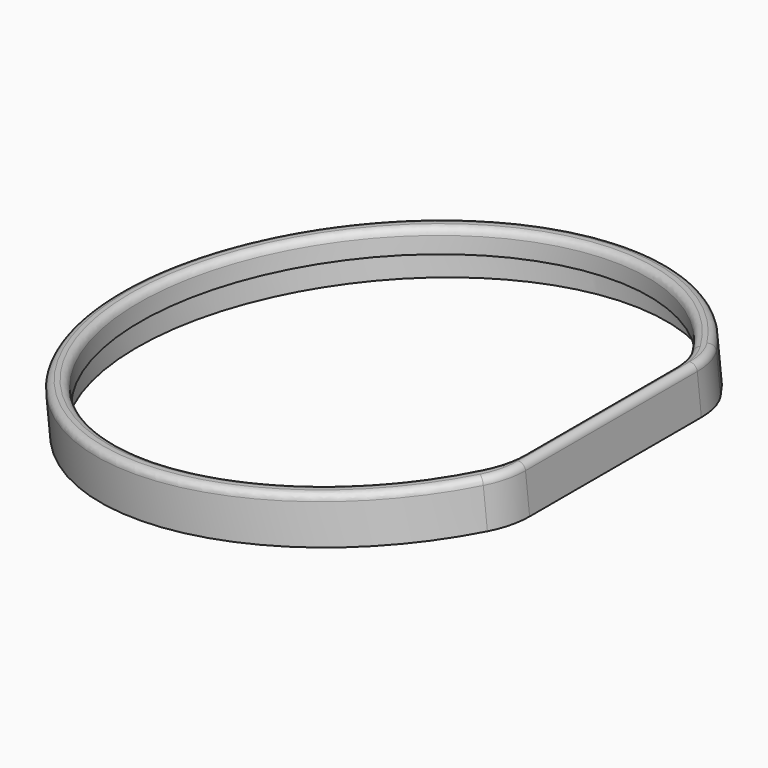
from build123d import *

# Parameters (mm, degrees)
F3_DEPTH     = 5
F4_DEPTH     = 5
F5_R         = 15
F6_T1_DEPTH  = 46.5006688801
F6_T3_DEPTH  = 40.6046915678
F6_T6_ANGLE  = 292.774155129
F6_T8_ANGLE  = 295.4108576805
F6_T10_ANGLE = 33.6129224355
F6_T12_ANGLE = 33.6129224355
F6_T14_ANGLE = 32.2945711597
F6_T16_ANGLE = 32.2945711597


# Not quite as in the source:
# - a fillet or chamfer that OpenCascade refuses, or shapes differently, is made with other operations: its cross-section is extruded or revolved along the edge and cut away or added


with BuildPart() as f3:
    # F2 (on line) → F3 (new body)
    with BuildSketch(Plane(origin=(-1.0990247565, 0, 10.4565220775), x_dir=(0.9945218954, 0, 0.1045284633), z_dir=(-0.1045284633, 0, 0.9945218954))):
        with BuildLine():
            add(Edge.make_bspline(
                [(48.8576467338, 27.4245012731), (32.937142649, 55.0146028399), (1, 55.0146028399)],
                knots=[3.6634544085, 3.6634544085, 3.6634544085, 4.7123889804, 4.7123889804, 4.7123889804], degree=2, weights=[1, 0.865590822, 1]))
            add(Edge.make_bspline(
                [(49.9774491412, 25.3853808752), (49.4391671103, 26.4167312826), (48.8576467338, 27.4245012731)],
                knots=[3.6211988828, 3.6211988828, 3.6211988828, 3.6634544085, 3.6634544085, 3.6634544085], degree=2, weights=[1, 0.9997768171, 1]))
            Line((49.9774491412, 25.3853808752), (49.9774491412, 27.409023648))
            ThreePointArc((49.9774491412, 27.409023648), (-57, 0), (49.9774491412, -27.409023648))
            Line((49.9774491412, -27.409023648), (49.9774491412, -25.3853808752))
            add(Edge.make_bspline(
                [(48.8576467338, -27.4245012731), (49.4391671103, -26.4167312826), (49.9774491412, -25.3853808752)],
                knots=[2.6197308987, 2.6197308987, 2.6197308987, 2.6619864244, 2.6619864244, 2.6619864244], degree=2, weights=[1, 0.9997768171, 1]))
            add(Edge.make_bspline(
                [(1, 55.0146028399), (-94.7155099565, 55.0146028399), (-46.785780422, -27.5486703855), (1.1439491125, -110.1119436109), (48.8576467338, -27.4245012731)],
                knots=[4.7123889804, 4.7123889804, 4.7123889804, 6.8076525931, 6.8076525931, 8.9029162059, 8.9029162059, 8.9029162059], degree=2, weights=[1, 0.4996238769, 1, 0.4996238769, 1]))
        make_face()
        with BuildLine():
            ThreePointArc((47.121873477, -24.2596174747), (-53, 0), (47.121873477, 24.2596174747))
            ThreePointArc((47.121873477, 24.2596174747), (48.0257660969, 22.4170870276), (48.8576467338, 20.540943397))
            Line((48.8576467338, 20.540943397), (48.8576467338, 27.4245012731))
            add(Edge.make_bspline(
                [(48.8576467338, 27.4245012731), (32.937142649, 55.0146028399), (1, 55.0146028399)],
                knots=[3.6634544085, 3.6634544085, 3.6634544085, 4.7123889804, 4.7123889804, 4.7123889804], degree=2, weights=[1, 0.865590822, 1]))
            add(Edge.make_bspline(
                [(1, 55.0146028399), (-94.7155099565, 55.0146028399), (-46.785780422, -27.5486703855), (1.1439491125, -110.1119436109), (48.8576467338, -27.4245012731)],
                knots=[4.7123889804, 4.7123889804, 4.7123889804, 6.8076525931, 6.8076525931, 8.9029162059, 8.9029162059, 8.9029162059], degree=2, weights=[1, 0.4996238769, 1, 0.4996238769, 1]))
            Line((48.8576467338, -27.4245012731), (48.8576467338, -20.540943397))
            ThreePointArc((48.8576467338, -20.540943397), (48.0257660969, -22.4170870276), (47.121873477, -24.2596174747))
        make_face()
        with BuildLine():
            ThreePointArc((48.8576467338, 20.540943397), (48.0257660969, 22.4170870276), (47.121873477, 24.2596174747))
            Line((47.121873477, 24.2596174747), (47.121873477, -24.2596174747))
            ThreePointArc((47.121873477, -24.2596174747), (48.0257660969, -22.4170870276), (48.8576467338, -20.540943397))
            Line((48.8576467338, -20.540943397), (48.8576467338, 20.540943397))
        make_face()
        with BuildLine():
            ThreePointArc((49.9774491412, 17.6424084902), (49.4387946891, 19.0998842848), (48.8576467338, 20.540943397))
            Line((48.8576467338, 20.540943397), (48.8576467338, -20.540943397))
            ThreePointArc((48.8576467338, -20.540943397), (49.4387946891, -19.0998842848), (49.9774491412, -17.6424084902))
            Line((49.9774491412, -17.6424084902), (49.9774491412, 17.6424084902))
        make_face()
        with BuildLine():
            Line((48.8576467338, 27.4245012731), (48.8576467338, 20.540943397))
            ThreePointArc((48.8576467338, 20.540943397), (49.4387946891, 19.0998842848), (49.9774491412, 17.6424084902))
            Line((49.9774491412, 17.6424084902), (49.9774491412, 25.3853808752))
            add(Edge.make_bspline(
                [(49.9774491412, 25.3853808752), (49.4391671103, 26.4167312826), (48.8576467338, 27.4245012731)],
                knots=[3.6211988828, 3.6211988828, 3.6211988828, 3.6634544085, 3.6634544085, 3.6634544085], degree=2, weights=[1, 0.9997768171, 1]))
        make_face()
        with BuildLine():
            ThreePointArc((49.9774491412, -17.6424084902), (49.4387946891, -19.0998842848), (48.8576467338, -20.540943397))
            Line((48.8576467338, -20.540943397), (48.8576467338, -27.4245012731))
            add(Edge.make_bspline(
                [(48.8576467338, -27.4245012731), (49.4391671103, -26.4167312826), (49.9774491412, -25.3853808752)],
                knots=[2.6197308987, 2.6197308987, 2.6197308987, 2.6619864244, 2.6619864244, 2.6619864244], degree=2, weights=[1, 0.9997768171, 1]))
            Line((49.9774491412, -25.3853808752), (49.9774491412, -17.6424084902))
        make_face()
    extrude(amount=F3_DEPTH)

    # F2 (on line) → F4 (join)
    with BuildSketch(Plane(origin=(-1.0990247565, 0, 10.4565220775), x_dir=(0.9945218954, 0, 0.1045284633), z_dir=(-0.1045284633, 0, 0.9945218954))):
        with BuildLine():
            add(Edge.make_bspline(
                [(48.8576467338, 27.4245012731), (32.937142649, 55.0146028399), (1, 55.0146028399)],
                knots=[3.6634544085, 3.6634544085, 3.6634544085, 4.7123889804, 4.7123889804, 4.7123889804], degree=2, weights=[1, 0.865590822, 1]))
            add(Edge.make_bspline(
                [(49.9774491412, 25.3853808752), (49.4391671103, 26.4167312826), (48.8576467338, 27.4245012731)],
                knots=[3.6211988828, 3.6211988828, 3.6211988828, 3.6634544085, 3.6634544085, 3.6634544085], degree=2, weights=[1, 0.9997768171, 1]))
            Line((49.9774491412, 25.3853808752), (49.9774491412, 27.409023648))
            ThreePointArc((49.9774491412, 27.409023648), (-57, 0), (49.9774491412, -27.409023648))
            Line((49.9774491412, -27.409023648), (49.9774491412, -25.3853808752))
            add(Edge.make_bspline(
                [(48.8576467338, -27.4245012731), (49.4391671103, -26.4167312826), (49.9774491412, -25.3853808752)],
                knots=[2.6197308987, 2.6197308987, 2.6197308987, 2.6619864244, 2.6619864244, 2.6619864244], degree=2, weights=[1, 0.9997768171, 1]))
            add(Edge.make_bspline(
                [(1, 55.0146028399), (-94.7155099565, 55.0146028399), (-46.785780422, -27.5486703855), (1.1439491125, -110.1119436109), (48.8576467338, -27.4245012731)],
                knots=[4.7123889804, 4.7123889804, 4.7123889804, 6.8076525931, 6.8076525931, 8.9029162059, 8.9029162059, 8.9029162059], degree=2, weights=[1, 0.4996238769, 1, 0.4996238769, 1]))
        make_face()
        with BuildLine():
            ThreePointArc((49.9774491412, -17.6424084902), (49.4387946891, -19.0998842848), (48.8576467338, -20.540943397))
            Line((48.8576467338, -20.540943397), (48.8576467338, -27.4245012731))
            add(Edge.make_bspline(
                [(48.8576467338, -27.4245012731), (49.4391671103, -26.4167312826), (49.9774491412, -25.3853808752)],
                knots=[2.6197308987, 2.6197308987, 2.6197308987, 2.6619864244, 2.6619864244, 2.6619864244], degree=2, weights=[1, 0.9997768171, 1]))
            Line((49.9774491412, -25.3853808752), (49.9774491412, -17.6424084902))
        make_face()
        with BuildLine():
            Line((48.8576467338, 27.4245012731), (48.8576467338, 20.540943397))
            ThreePointArc((48.8576467338, 20.540943397), (49.4387946891, 19.0998842848), (49.9774491412, 17.6424084902))
            Line((49.9774491412, 17.6424084902), (49.9774491412, 25.3853808752))
            add(Edge.make_bspline(
                [(49.9774491412, 25.3853808752), (49.4391671103, 26.4167312826), (48.8576467338, 27.4245012731)],
                knots=[3.6211988828, 3.6211988828, 3.6211988828, 3.6634544085, 3.6634544085, 3.6634544085], degree=2, weights=[1, 0.9997768171, 1]))
        make_face()
        with BuildLine():
            ThreePointArc((49.9774491412, 17.6424084902), (49.4387946891, 19.0998842848), (48.8576467338, 20.540943397))
            Line((48.8576467338, 20.540943397), (48.8576467338, -20.540943397))
            ThreePointArc((48.8576467338, -20.540943397), (49.4387946891, -19.0998842848), (49.9774491412, -17.6424084902))
            Line((49.9774491412, -17.6424084902), (49.9774491412, 17.6424084902))
        make_face()
    extrude(amount=-F4_DEPTH)

    # F5
    f5_edges = [f3.edges().sort_by_distance(p)[0] for p in [
        (45.503389, 24.259617, 17.868404),
        (47.752296, 27.424501, 13.077232),
        (48.604643, -27.409024, 15.680588),
        (48.604643, 27.409024, 15.680588),
        (47.752296, -27.424501, 13.077232),
        (45.503389, -24.259617, 17.868404),
    ]]
    fillet(f5_edges, radius=F5_R)

    # F6: fillet of radius 1.5 on 8 edges, made by hand

    # F6_s2 → F6_t1 (cut)
    with BuildSketch(Plane.XZ.offset(-23.25033444)):
        with BuildLine():
            ThreePointArc((48.2387930677, 19.161414668), (47.6909908112, 20.1703409153), (46.5902175297, 20.4964048162))
            Line((46.5902175297, 20.4964048162), (48.0820003728, 20.6531975111))
            Line((48.0820003728, 20.6531975111), (48.2387930677, 19.161414668))
        make_face()
    extrude(amount=F6_T1_DEPTH, mode=Mode.SUBTRACT)

    # F6_s4 → F6_t3 (cut)
    with BuildSketch(Plane.XZ.offset(-20.3023457839)):
        with BuildLine():
            ThreePointArc((46.7338506938, 20.5115012701), (45.7249244466, 19.9636990136), (45.3988605457, 18.8629257321))
            Line((45.3988605457, 18.8629257321), (45.2420678508, 20.3547085752))
            Line((45.2420678508, 20.3547085752), (46.7338506938, 20.5115012701))
        make_face()
    extrude(amount=F6_T3_DEPTH, mode=Mode.SUBTRACT)

    # F6_s5 → F6_t6 (revolve, cut)
    with BuildSketch(Plane(origin=(0, 0, 0), x_dir=(0.8341941601, 0.5514708544, 0), z_dir=(0.5505468256, -0.8327964081, 0.0578648031))):
        with BuildLine():
            ThreePointArc((53.9358200017, 20.2944629237), (55.0307493385, 19.9492829243), (55.5609021792, 18.930971847))
            Line((55.5609021792, 18.930971847), (55.4301066288, 20.4252584742))
            Line((55.4301066288, 20.4252584742), (53.9358200017, 20.2944629237))
        make_face()
    revolve(axis=Axis((-1.6216670728, 0, 15.4291315543), (-0.1045284633, 0, 0.9945218954)), revolution_arc=F6_T6_ANGLE, mode=Mode.SUBTRACT)

    # F6_s7 → F6_t8 (revolve, cut)
    with BuildSketch(Plane(origin=(0, 0, 0), x_dir=(-0.8466337525, 0.5321759946, 0), z_dir=(0.5313454581, 0.8453124599, 0.055846658))):
        with BuildLine():
            ThreePointArc((-52.9132065092, 20.2763527671), (-51.8955883279, 19.7448711382), (-51.5518378751, 18.6494921577))
            Line((-51.5518378751, 18.6494921577), (-51.4190918875, 20.1436067794))
            Line((-51.4190918875, 20.1436067794), (-52.9132065092, 20.2763527671))
        make_face()
    revolve(axis=Axis((-1.6216670728, 0, 15.4291315543), (0.1045284633, 0, -0.9945218954)), revolution_arc=F6_T8_ANGLE, mode=Mode.SUBTRACT)

    # F6_s9 → F6_t10 (revolve, cut)
    with BuildSketch(Plane.XZ.offset(23.25033444)):
        with BuildLine():
            ThreePointArc((46.5902175297, 20.4964048162), (47.6909908112, 20.1703409153), (48.2387930677, 19.161414668))
            Line((48.2387930677, 19.161414668), (48.0820003728, 20.6531975111))
            Line((48.0820003728, 20.6531975111), (46.5902175297, 20.4964048162))
        make_face()
    revolve(axis=Axis((33.1641719422, -23.25033444, 19.0852705621), (0.1045284633, 0, -0.9945218954)), revolution_arc=F6_T10_ANGLE, mode=Mode.SUBTRACT)

    # F6_s11 → F6_t12 (revolve, cut)
    with BuildSketch(Plane.XZ.offset(-23.25033444)):
        with BuildLine():
            ThreePointArc((46.5902175297, 20.4964048162), (47.6909908112, 20.1703409153), (48.2387930677, 19.161414668))
            Line((48.2387930677, 19.161414668), (48.0820003728, 20.6531975111))
            Line((48.0820003728, 20.6531975111), (46.5902175297, 20.4964048162))
        make_face()
    revolve(axis=Axis((33.1641719422, 23.25033444, 19.0852705621), (-0.1045284633, 0, 0.9945218954)), revolution_arc=F6_T12_ANGLE, mode=Mode.SUBTRACT)

    # F6_s13 → F6_t14 (revolve, cut)
    with BuildSketch(Plane.XZ.offset(20.3023457839)):
        with BuildLine():
            ThreePointArc((46.7338506938, 20.5115012701), (45.7249244466, 19.9636990136), (45.3988605457, 18.8629257321))
            Line((45.3988605457, 18.8629257321), (45.2420678508, 20.3547085752))
            Line((45.2420678508, 20.3547085752), (46.7338506938, 20.5115012701))
        make_face()
    revolve(axis=Axis((30.3242394203, -20.3023457839, 18.7867816262), (0.1045284633, 0, -0.9945218954)), revolution_arc=F6_T14_ANGLE, mode=Mode.SUBTRACT)

    # F6_s15 → F6_t16 (revolve, cut)
    with BuildSketch(Plane.XZ.offset(-20.3023457839)):
        with BuildLine():
            ThreePointArc((46.7338506938, 20.5115012701), (45.7249244466, 19.9636990136), (45.3988605457, 18.8629257321))
            Line((45.3988605457, 18.8629257321), (45.2420678508, 20.3547085752))
            Line((45.2420678508, 20.3547085752), (46.7338506938, 20.5115012701))
        make_face()
    revolve(axis=Axis((30.3242394203, 20.3023457839, 18.7867816262), (-0.1045284633, 0, 0.9945218954)), revolution_arc=F6_T16_ANGLE, mode=Mode.SUBTRACT)


solid = f3.part
